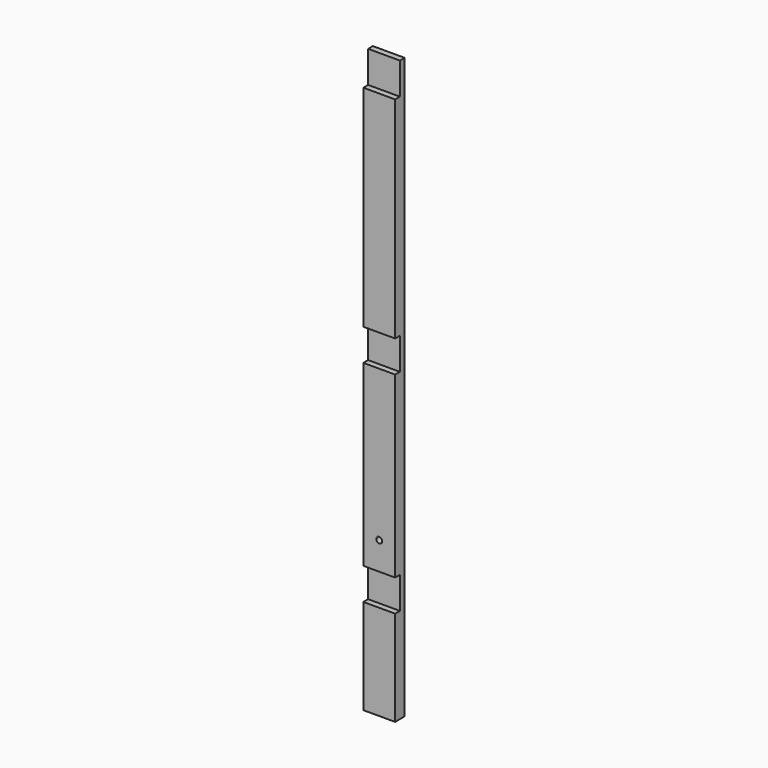
from build123d import *

# Parameters (mm, degrees)
F0_W     = 50.8
F0_H     = 19.05
F1_DEPTH = 927.1
F2_W     = 122.43557321
F2_H     = 50.8
F2_W_2   = 343.1604206562
F2_W_3   = 264.5317912102
F3_DEPTH = 25.4
F4_R     = 4.7625
F5_DEPTH = 25.4


# Not quite as in the source:
# - a feature names something its author has since deleted; it is built from what else it names


with BuildPart() as f1:
    # F0 (on Top) → F1 (new body)
    with BuildSketch(Plane.XY):
        Rectangle(F0_W, F0_H)
    extrude(amount=F1_DEPTH)

    # F2 (on Front) → F3 (cut)
    with BuildSketch(Plane.XZ):
        with Locations((22.4465244144, 177.8)):
            Rectangle(F2_W, F2_H)
        with Locations((-38.7818217278, 901.7)):
            Rectangle(F2_W_2, F2_H)
        with Locations((-47.6498156786, 514.35)):
            Rectangle(F2_W_3, F2_H)
    extrude(amount=F3_DEPTH, mode=Mode.SUBTRACT)

    # F4 (on Front) → F5 (cut)
    with BuildSketch(Plane.XZ):
        with Locations((0, 247.65)):
            Circle(F4_R)
    extrude(amount=F5_DEPTH, mode=Mode.SUBTRACT)


solid = f1.part
